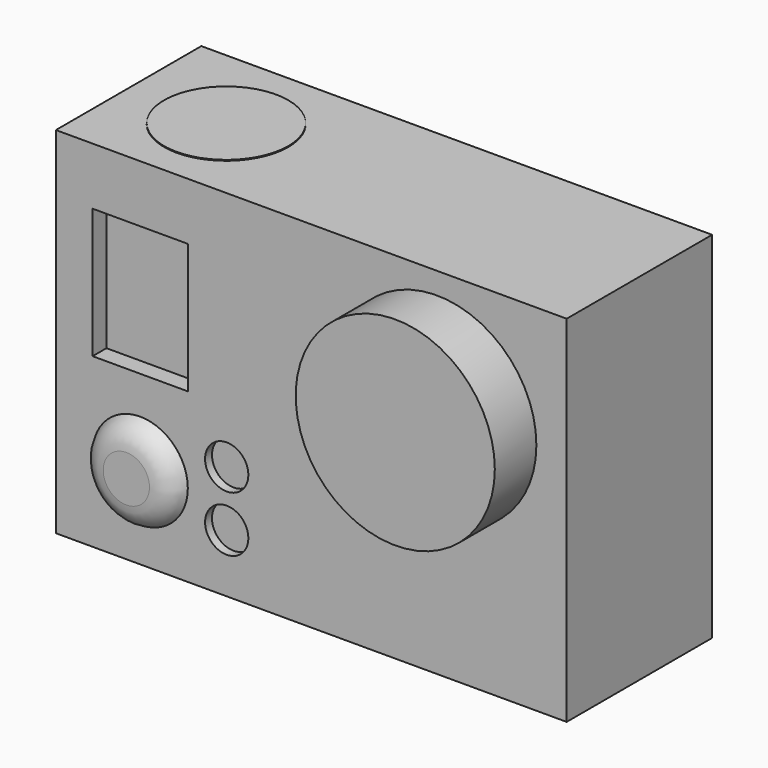
from build123d import *

# Parameters (mm, degrees)
F0_W      = 59
F0_H      = 41
F1_DEPTH  = 21
F2_R      = 11.5
F3_DEPTH  = 6
F2_W      = 11
F2_H      = 15
F4_DEPTH  = 2
F2_R_2    = 5.5
F5_DEPTH  = 2
F2_R_3    = 2.5
F7_DEPTH  = 1
F8_R      = 2.913941294
F9_DEPTH  = 1
F10_R     = 7.1742199979
F11_DEPTH = 0.1


# Not quite as in the source:
# - a fillet or chamfer that OpenCascade refuses, or shapes differently, is made with other operations: its cross-section is extruded or revolved along the edge and cut away or added
# - a feature of the source that left no trace in its solid (it failed there, or was rolled back) is left out


with BuildPart() as f1:
    # F0 (on Front) → F1 (new body)
    with BuildSketch(Plane.XZ):
        with Locations((-29.5, 20.5)):
            Rectangle(F0_W, F0_H)
    extrude(amount=F1_DEPTH)

    # F2 (on face) → F3 (join)
    with BuildSketch(Plane.XZ.offset(21)):
        with Locations((-15, 27)):
            Circle(F2_R)
    extrude(amount=F3_DEPTH)

    # F2 (on face) → F4 (cut)
    with BuildSketch(Plane.XZ.offset(21)):
        with Locations((-49.2600723803, 26.8833857775)):
            Rectangle(F2_W, F2_H)
    extrude(amount=-F4_DEPTH, mode=Mode.SUBTRACT)

    # F2 (on face) → F5 (join)
    with BuildSketch(Plane.XZ.offset(21)):
        with Locations((-49.2600723803, 9.5262574032)):
            Circle(F2_R_2)
    extrude(amount=F5_DEPTH)

    # F6: fillet of radius 3 on 1 edges, made by hand

    # F6_s1 → F6_t2 (revolve, cut)
    with BuildSketch(Plane.XY.offset(9.5262574032)):
        with BuildLine():
            ThreePointArc((-43.7600723803, -21), (-44.8564486975, -22.4494897428), (-46.5884995051, -23))
            Line((-46.5884995051, -23), (-43.7600723803, -23))
            Line((-43.7600723803, -23), (-43.7600723803, -21))
        make_face()
    revolve(axis=Axis((-49.2600723803, -23, 9.5262574032), (0, -1, 0)), mode=Mode.SUBTRACT)

    # F2 (on face) → F7 (cut)
    with BuildSketch(Plane.XZ.offset(21)):
        with Locations((-39.2693579197, 13.1571451202)):
            Circle(F2_R_3)
        with Locations((-39.2693579197, 6.7239077762)):
            Circle(F2_R_3)
    extrude(amount=-F7_DEPTH, mode=Mode.SUBTRACT)

    # F8 (on face) → F9 (join)
    with BuildSketch(Plane(origin=(-59, 0, 0), x_dir=(0, -1, 0), z_dir=(-1, 0, 0))):
        with Locations((11.0362954438, 7.4682990089)):
            Circle(F8_R)
    extrude(amount=F9_DEPTH)

    # F10 (on face) → F11 (join)
    with BuildSketch(Plane.XY.offset(41)):
        with Locations((-47.7264709771, -10.5)):
            Circle(F10_R)
    extrude(amount=F11_DEPTH)


solid = f1.part
